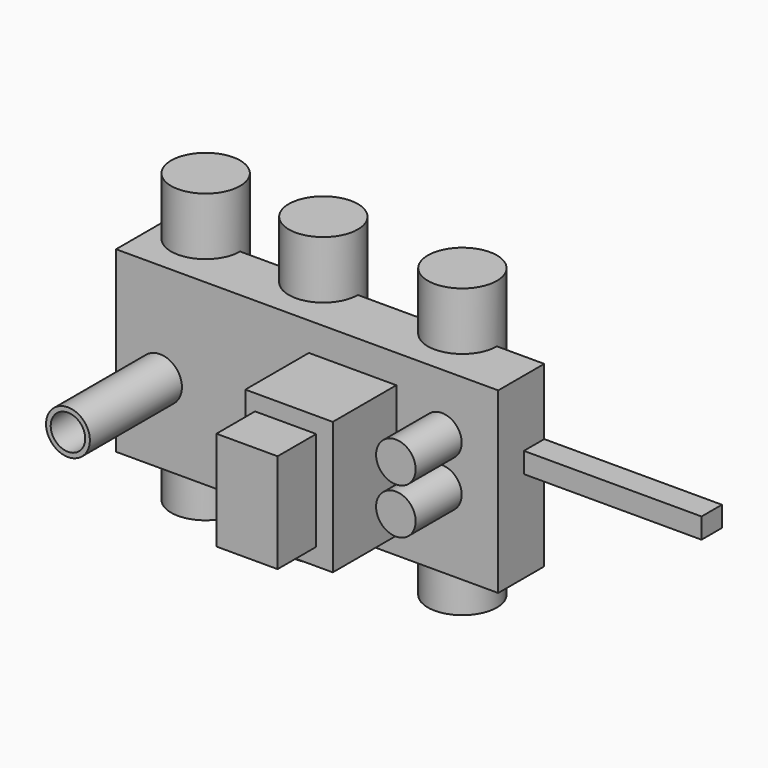
from build123d import *

# Parameters (mm, degrees)
F0_W      = 84.3690671027
F0_H      = 39.3722336739
F1_DEPTH  = 12.7
F4_W      = 5.6246062741
F4_H      = 4.5193769038
F5_DEPTH  = 61.722
F6_R      = 7.62
F7_DEPTH  = 63.5
F8_R      = 4.83847219
F9_DEPTH  = 38.1
F11_D     = 7.62
F13_W     = 34.8725486547
F13_H     = 29.2479414493
F14_DEPTH = 19.304
F16_D     = 10.16
F17_W     = 13.4990508668
F17_H     = 21.9359584153
F18_DEPTH = 40.894
F19_R     = 4.3749146568
F19_R_2   = 4.3688
F20_DEPTH = 25.4


# Not quite as in the source:
# - the program builds the solid bodies; features that only make, move or delete a surface that nothing else refers to are left out


with BuildPart() as f1:
    # F0 (on Front) → F1 (new body)
    with BuildSketch(Plane.XZ):
        with Locations((-19.6861159056, 31.0759413987)):
            Rectangle(F0_W, F0_H)
    extrude(amount=F1_DEPTH)

    # F4 (on Right) → F5 (join)
    with BuildSketch(Plane.YZ):
        with Locations((-2.812303137, 33.8783953339)):
            Rectangle(F4_W, F4_H)
    extrude(amount=F5_DEPTH)

    # F6 (on Top) → F7 (join)
    with BuildSketch(Plane.XY):
        with Locations((-52.2527975643, 0)):
            Circle(F6_R)
        with Locations((-26.2740052346, 0)):
            Circle(F6_R)
        with Locations((4.4282053044, 0)):
            Circle(F6_R)
    extrude(amount=F7_DEPTH)

    # F8 (on Front) → F9 (join)
    with BuildSketch(Plane.XZ):
        with Locations((-52.1682091057, 28.6854822189)):
            Circle(F8_R)
    extrude(amount=F9_DEPTH)

    # F11 (through all)
    with Locations(Plane.XZ.offset(38.1)):
        with Locations((-52.1682091057, 28.6854822189)):
            Hole(F11_D / 2)

    # F13 (on Right) → F14 (join)
    with BuildSketch(Plane.YZ):
        with Locations((-12.7959763631, 29.8289656639)):
            Rectangle(F13_W, F13_H)
    extrude(amount=-F14_DEPTH)

    # F16 (through all)
    with Locations(Plane(origin=(0, 4.6402979642, 0), x_dir=(-1, 0, 0), z_dir=(0, 1, 0))):
        with Locations((10.4055171832, 30.513478443)):
            Hole(F16_D / 2)

    # F17 (on Front) → F18 (join)
    with BuildSketch(Plane.XZ):
        with Locations((-10.4055190459, 29.9460180104)):
            Rectangle(F17_W, F17_H)
    extrude(amount=F18_DEPTH)

    # F19 (on Front) → F20 (join)
    with BuildSketch(Plane.XZ):
        with Locations((10.0624421611, 27.8602354228)):
            Circle(F19_R)
        with Locations((10.0624421611, 37.9722304642)):
            Circle(F19_R_2)
    extrude(amount=F20_DEPTH)


solid = f1.part
